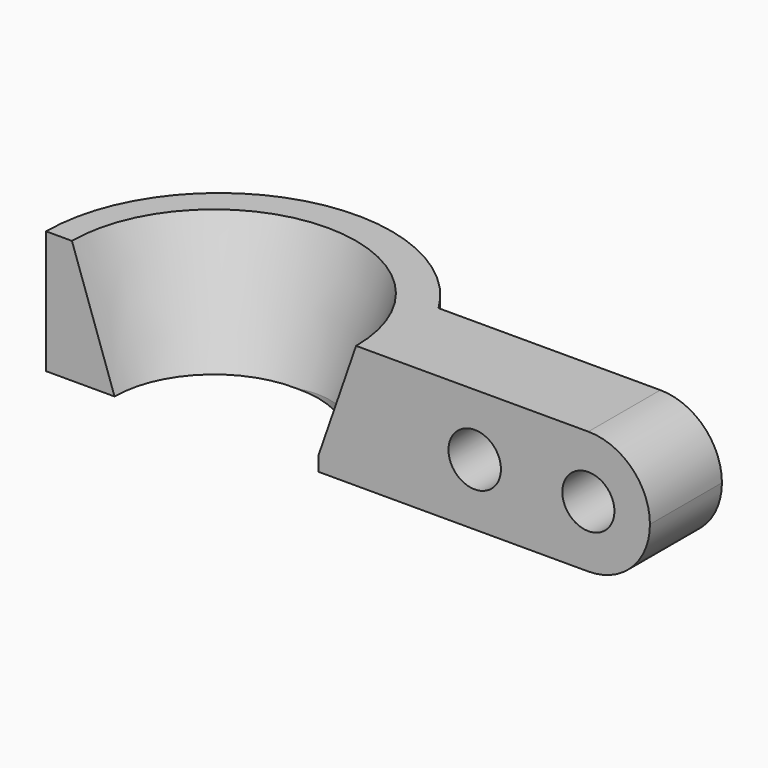
from build123d import *

# Parameters (mm, degrees)
F1_DEPTH = 52
F2_R     = 11.0802059784
F2_R_2   = 11
F3_DEPTH = 51.6
F4_R     = 25.99999


# Not quite as in the source:
# - a fillet or chamfer is up to 0.001 mm smaller than in the source, because OpenCascade refuses the exact size


with BuildPart() as f1:
    # F0 (on Top) → F1 (new body)
    with BuildSketch(Plane.XY):
        with BuildLine():
            Line((109, 38), (-10.670231831, 38))
            ThreePointArc((-10.670231831, 38), (-92.7348286497, 70.2818364741), (-146, 0))
            Line((-146, 0), (-115, 0))
            ThreePointArc((-115, 0), (-73, 42), (-31, 0))
            Line((-31, 0), (109, 0))
            Line((109, 0), (109, 38))
        make_face()
    extrude(amount=F1_DEPTH)

    # F2 (on face) → F3 (cut)
    with BuildSketch(Plane.XZ):
        with Locations((35, 26)):
            Circle(F2_R)
        with Locations((83, 26)):
            Circle(F2_R_2)
    extrude(amount=-F3_DEPTH, mode=Mode.SUBTRACT)

    # F4 (radius 26 in the source; OpenCascade refuses exactly that, so slightly less here)
    f4_edges = [f1.edges().sort_by_distance(p)[0] for p in [
        (109, 19, 52),
        (109, 19, 0),
    ]]
    fillet(f4_edges, radius=F4_R)

    # F5 (on face) → F6 (revolve, cut)
    with BuildSketch(Plane.XZ):
        Polygon((-75.0884139538, 52), (-135.0884139538, 52), (-117.0884139538, 0), (-75.0884139538, 0), align=None)
    revolve(axis=Axis((-75.0884139538, 0, 26), (0, 0, 1)), mode=Mode.SUBTRACT)


solid = f1.part
